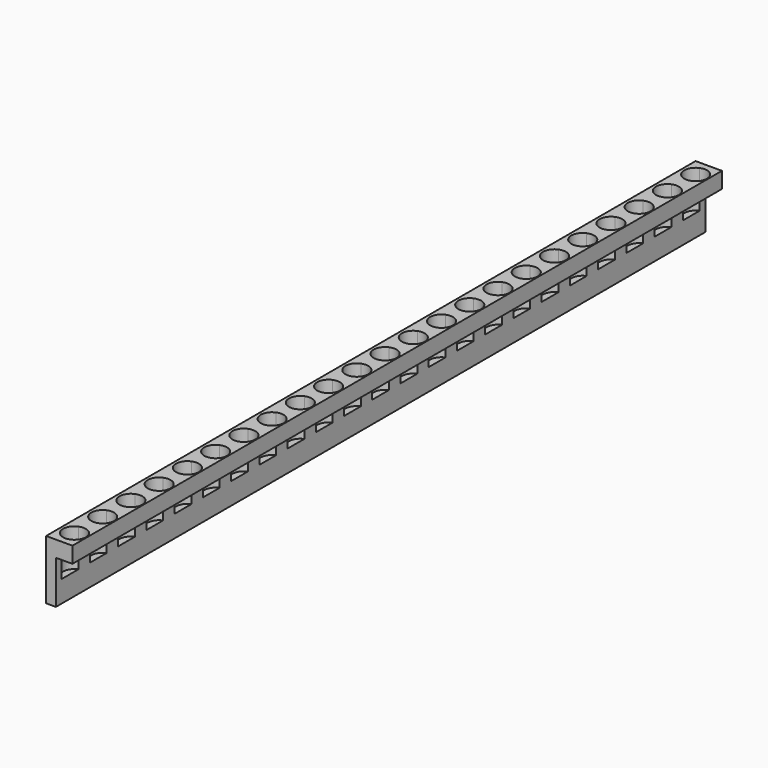
from build123d import *
from build123d import SkipClean  # not in build123d's __all__

# Parameters (mm, degrees)
F1_DEPTH = 4.318
F2_DEPTH = 4.318
F3_DEPTH = 5.842
F4_W     = 2.6416
F4_H     = 222.25
F5_DEPTH = 5.842
F6_DEPTH = 0.00508
F7_DEPTH = 3.19786


# Not quite as in the source:
# - after a boolean that leaves OpenCascade's solid faulty, fix() repairs it


with BuildPart() as f1:
    # F0 (on Top) → F1 (new body)
    with BuildSketch(Plane.XY):
        with BuildLine():
            Line((-21.6095393037, 173.5015366077), (-26.0799393037, 173.5015366077))
            Line((-26.0799393037, 173.5015366077), (-26.0799393037, 168.3720872764))
            ThreePointArc((-26.0799393037, 168.3720872764), (-23.1852887823, 168.1025078341), (-21.8103172985, 165.5410379171))
            ThreePointArc((-21.8103172985, 165.5410379171), (-23.1852887823, 162.9795680002), (-26.0799393037, 162.7099885579))
            Line((-26.0799393037, 162.7099885579), (-26.0799393037, 158.8512725119))
            ThreePointArc((-26.0799393037, 158.8512725119), (-23.1852887823, 158.5816930696), (-21.8103172985, 156.0202231526))
            ThreePointArc((-21.8103172985, 156.0202231526), (-23.1852887823, 153.4587532357), (-26.0799393037, 153.1891737934))
            Line((-26.0799393037, 153.1891737934), (-26.0799393037, 149.3262725119))
            ThreePointArc((-26.0799393037, 149.3262725119), (-23.1852887823, 149.0566930696), (-21.8103172985, 146.4952231526))
            ThreePointArc((-21.8103172985, 146.4952231526), (-23.1852887823, 143.9337532357), (-26.0799393037, 143.6641737934))
            Line((-26.0799393037, 143.6641737934), (-26.0799393037, 139.8012725119))
            ThreePointArc((-26.0799393037, 139.8012725119), (-23.1852887823, 139.5316930696), (-21.8103172985, 136.9702231526))
            ThreePointArc((-21.8103172985, 136.9702231526), (-23.1852887823, 134.4087532357), (-26.0799393037, 134.1391737934))
            Line((-26.0799393037, 134.1391737934), (-26.0799393037, 130.2762725119))
            ThreePointArc((-26.0799393037, 130.2762725119), (-23.1852887823, 130.0066930696), (-21.8103172985, 127.4452231526))
            ThreePointArc((-21.8103172985, 127.4452231526), (-23.1852887823, 124.8837532357), (-26.0799393037, 124.6141737934))
            Line((-26.0799393037, 124.6141737934), (-26.0799393037, 120.7512725119))
            ThreePointArc((-26.0799393037, 120.7512725119), (-23.1852887823, 120.4816930696), (-21.8103172985, 117.9202231526))
            ThreePointArc((-21.8103172985, 117.9202231526), (-23.1852887823, 115.3587532357), (-26.0799393037, 115.0891737934))
            Line((-26.0799393037, 115.0891737934), (-26.0799393037, 111.2262725119))
            ThreePointArc((-26.0799393037, 111.2262725119), (-23.1852887823, 110.9566930696), (-21.8103172985, 108.3952231526))
            ThreePointArc((-21.8103172985, 108.3952231526), (-23.1852887823, 105.8337532357), (-26.0799393037, 105.5641737934))
            Line((-26.0799393037, 105.5641737934), (-26.0799393037, 101.7012725119))
            ThreePointArc((-26.0799393037, 101.7012725119), (-23.1852887823, 101.4316930696), (-21.8103172985, 98.8702231526))
            ThreePointArc((-21.8103172985, 98.8702231526), (-23.1852887823, 96.3087532357), (-26.0799393037, 96.0391737934))
            Line((-26.0799393037, 96.0391737934), (-26.0799393037, 92.1762725119))
            ThreePointArc((-26.0799393037, 92.1762725119), (-23.1852887823, 91.9066930696), (-21.8103172985, 89.3452231526))
            ThreePointArc((-21.8103172985, 89.3452231526), (-23.1852887823, 86.7837532357), (-26.0799393037, 86.5141737934))
            Line((-26.0799393037, 86.5141737934), (-26.0799393037, 82.6512725119))
            ThreePointArc((-26.0799393037, 82.6512725119), (-23.1852887823, 82.3816930696), (-21.8103172985, 79.8202231526))
            ThreePointArc((-21.8103172985, 79.8202231526), (-23.1852887823, 77.2587532357), (-26.0799393037, 76.9891737934))
            Line((-26.0799393037, 76.9891737934), (-26.0799393037, 73.1374398831))
            ThreePointArc((-26.0799393037, 73.1374398831), (-23.1852887823, 72.8678604408), (-21.8103172985, 70.3063905239))
            ThreePointArc((-21.8103172985, 70.3063905239), (-23.1852887823, 67.744920607), (-26.0799393037, 67.4753411647))
            Line((-26.0799393037, 67.4753411647), (-26.0799393037, 63.6124425594))
            ThreePointArc((-26.0799393037, 63.6124425594), (-23.1852887823, 63.3428631171), (-21.8103172985, 60.7813932002))
            ThreePointArc((-21.8103172985, 60.7813932002), (-23.1852887823, 58.2199232832), (-26.0799393037, 57.9503438409))
            Line((-26.0799393037, 57.9503438409), (-26.0799393037, 54.0874415103))
            ThreePointArc((-26.0799393037, 54.0874415103), (-23.1852887823, 53.817862068), (-21.8103172985, 51.2563921511))
            ThreePointArc((-21.8103172985, 51.2563921511), (-23.1852887823, 48.6949222342), (-26.0799393037, 48.4253427919))
            Line((-26.0799393037, 48.4253427919), (-26.0799393037, 44.5624441866))
            ThreePointArc((-26.0799393037, 44.5624441866), (-23.1852887823, 44.2928647443), (-21.8103172985, 41.7313948274))
            ThreePointArc((-21.8103172985, 41.7313948274), (-23.1852887823, 39.1699249104), (-26.0799393037, 38.9003454681))
            Line((-26.0799393037, 38.9003454681), (-26.0799393037, 35.0374431376))
            ThreePointArc((-26.0799393037, 35.0374431376), (-23.1852887823, 34.7678636953), (-21.8103172985, 32.2063937783))
            ThreePointArc((-21.8103172985, 32.2063937783), (-23.1852887823, 29.6449238614), (-26.0799393037, 29.3753444191))
            Line((-26.0799393037, 29.3753444191), (-26.0799393037, 25.5124439512))
            ThreePointArc((-26.0799393037, 25.5124439512), (-23.1852887823, 25.2428645089), (-21.8103172985, 22.6813945919))
            ThreePointArc((-21.8103172985, 22.6813945919), (-23.1852887823, 20.119924675), (-26.0799393037, 19.8503452327))
            Line((-26.0799393037, 19.8503452327), (-26.0799393037, 15.9874438334))
            ThreePointArc((-26.0799393037, 15.9874438334), (-23.1852887823, 15.7178643911), (-21.8103172985, 13.1563944742))
            ThreePointArc((-21.8103172985, 13.1563944742), (-23.1852887823, 10.5949245573), (-26.0799393037, 10.325345115))
            Line((-26.0799393037, 10.325345115), (-26.0799393037, 6.4624434829))
            ThreePointArc((-26.0799393037, 6.4624434829), (-23.1852887823, 6.1928640406), (-21.8103172985, 3.6313941237))
            ThreePointArc((-21.8103172985, 3.6313941237), (-23.1852887823, 1.0699242067), (-26.0799393037, 0.8003447644))
            Line((-26.0799393037, 0.8003447644), (-26.0799393037, -3.0625568677))
            ThreePointArc((-26.0799393037, -3.0625568677), (-23.1852887823, -3.33213631), (-21.8103172985, -5.8936062269))
            ThreePointArc((-21.8103172985, -5.8936062269), (-23.1852887823, -8.4550761438), (-26.0799393037, -8.7246555861))
            Line((-26.0799393037, -8.7246555861), (-26.0799393037, -12.5809180524))
            ThreePointArc((-26.0799393037, -12.5809180524), (-23.1852887823, -12.8504974947), (-21.8103172985, -15.4119674116))
            ThreePointArc((-21.8103172985, -15.4119674116), (-23.1852887823, -17.9734373286), (-26.0799393037, -18.2430167709))
            Line((-26.0799393037, -18.2430167709), (-26.0799393037, -22.1085814592))
            ThreePointArc((-26.0799393037, -22.1085814592), (-23.1860931255, -22.3777536514), (-21.8114210892, -24.9384324998))
            ThreePointArc((-21.8114210892, -24.9384324998), (-23.1860931255, -27.4991113482), (-26.0799393037, -27.7682835404))
            Line((-26.0799393037, -27.7682835404), (-26.0799393037, -31.6266121611))
            ThreePointArc((-26.0799393037, -31.6266121611), (-23.1857640907, -31.8959509553), (-21.8109695623, -34.4569534063))
            ThreePointArc((-21.8109695623, -34.4569534063), (-23.1857640907, -37.0179558574), (-26.0799393037, -37.2872946516))
            Line((-26.0799393037, -37.2872946516), (-26.0799393037, -41.149786583))
            ThreePointArc((-26.0799393037, -41.149786583), (-23.1818467711, -41.4211080967), (-21.8055935227, -43.9859633923))
            ThreePointArc((-21.8055935227, -43.9859633923), (-23.1818467711, -46.5508186878), (-26.0799393037, -46.8221402015))
            Line((-26.0799393037, -46.8221402015), (-26.0799393037, -47.7885268629))
            Line((-26.0799393037, -47.7885268629), (-26.0799393037, -48.7484633923))
            Line((-26.0799393037, -48.7484633923), (-21.6095393037, -48.7484633923))
            Line((-21.6095393037, -48.7484633923), (-21.6095393037, 173.5015366077))
        make_face()
    extrude(amount=F1_DEPTH)

    # F0 (on Top) → F2 (join)
    with BuildSketch(Plane.XY):
        with BuildLine():
            Line((-26.0799393037, 173.5015366077), (-28.7215393037, 173.5015366077))
            Line((-28.7215393037, 173.5015366077), (-28.7215393037, -48.7484633923))
            Line((-28.7215393037, -48.7484633923), (-26.0799393037, -48.7484633923))
            Line((-26.0799393037, -48.7484633923), (-26.0799393037, -47.7885268629))
            Line((-26.0799393037, -47.7885268629), (-26.0799393037, -46.8221402015))
            ThreePointArc((-26.0799393037, -46.8221402015), (-27.9618410743, -43.9859633923), (-26.0799393037, -41.149786583))
            Line((-26.0799393037, -41.149786583), (-26.0799393037, -37.2872946516))
            ThreePointArc((-26.0799393037, -37.2872946516), (-27.9564650347, -34.4569534063), (-26.0799393037, -31.6266121611))
            Line((-26.0799393037, -31.6266121611), (-26.0799393037, -27.7682835404))
            ThreePointArc((-26.0799393037, -27.7682835404), (-27.9560135078, -24.9384324998), (-26.0799393037, -22.1085814592))
            Line((-26.0799393037, -22.1085814592), (-26.0799393037, -18.2430167709))
            ThreePointArc((-26.0799393037, -18.2430167709), (-27.9571172985, -15.4119674116), (-26.0799393037, -12.5809180524))
            Line((-26.0799393037, -12.5809180524), (-26.0799393037, -8.7246555861))
            ThreePointArc((-26.0799393037, -8.7246555861), (-27.9571172985, -5.8936062269), (-26.0799393037, -3.0625568677))
            Line((-26.0799393037, -3.0625568677), (-26.0799393037, 0.8003447644))
            ThreePointArc((-26.0799393037, 0.8003447644), (-27.9571172985, 3.6313941237), (-26.0799393037, 6.4624434829))
            Line((-26.0799393037, 6.4624434829), (-26.0799393037, 10.325345115))
            ThreePointArc((-26.0799393037, 10.325345115), (-27.9571172985, 13.1563944742), (-26.0799393037, 15.9874438334))
            Line((-26.0799393037, 15.9874438334), (-26.0799393037, 19.8503452327))
            ThreePointArc((-26.0799393037, 19.8503452327), (-27.9571172985, 22.6813945919), (-26.0799393037, 25.5124439512))
            Line((-26.0799393037, 25.5124439512), (-26.0799393037, 29.3753444191))
            ThreePointArc((-26.0799393037, 29.3753444191), (-27.9571172985, 32.2063937783), (-26.0799393037, 35.0374431376))
            Line((-26.0799393037, 35.0374431376), (-26.0799393037, 38.9003454681))
            ThreePointArc((-26.0799393037, 38.9003454681), (-27.9571172985, 41.7313948274), (-26.0799393037, 44.5624441866))
            Line((-26.0799393037, 44.5624441866), (-26.0799393037, 48.4253427919))
            ThreePointArc((-26.0799393037, 48.4253427919), (-27.9571172985, 51.2563921511), (-26.0799393037, 54.0874415103))
            Line((-26.0799393037, 54.0874415103), (-26.0799393037, 57.9503438409))
            ThreePointArc((-26.0799393037, 57.9503438409), (-27.9571172985, 60.7813932002), (-26.0799393037, 63.6124425594))
            Line((-26.0799393037, 63.6124425594), (-26.0799393037, 67.4753411647))
            ThreePointArc((-26.0799393037, 67.4753411647), (-27.9571172985, 70.3063905239), (-26.0799393037, 73.1374398831))
            Line((-26.0799393037, 73.1374398831), (-26.0799393037, 76.9891737934))
            ThreePointArc((-26.0799393037, 76.9891737934), (-27.9571172985, 79.8202231526), (-26.0799393037, 82.6512725119))
            Line((-26.0799393037, 82.6512725119), (-26.0799393037, 86.5141737934))
            ThreePointArc((-26.0799393037, 86.5141737934), (-27.9571172985, 89.3452231526), (-26.0799393037, 92.1762725119))
            Line((-26.0799393037, 92.1762725119), (-26.0799393037, 96.0391737934))
            ThreePointArc((-26.0799393037, 96.0391737934), (-27.9571172985, 98.8702231526), (-26.0799393037, 101.7012725119))
            Line((-26.0799393037, 101.7012725119), (-26.0799393037, 105.5641737934))
            ThreePointArc((-26.0799393037, 105.5641737934), (-27.9571172985, 108.3952231526), (-26.0799393037, 111.2262725119))
            Line((-26.0799393037, 111.2262725119), (-26.0799393037, 115.0891737934))
            ThreePointArc((-26.0799393037, 115.0891737934), (-27.9571172985, 117.9202231526), (-26.0799393037, 120.7512725119))
            Line((-26.0799393037, 120.7512725119), (-26.0799393037, 124.6141737934))
            ThreePointArc((-26.0799393037, 124.6141737934), (-27.9571172985, 127.4452231526), (-26.0799393037, 130.2762725119))
            Line((-26.0799393037, 130.2762725119), (-26.0799393037, 134.1391737934))
            ThreePointArc((-26.0799393037, 134.1391737934), (-27.9571172985, 136.9702231526), (-26.0799393037, 139.8012725119))
            Line((-26.0799393037, 139.8012725119), (-26.0799393037, 143.6641737934))
            ThreePointArc((-26.0799393037, 143.6641737934), (-27.9571172985, 146.4952231526), (-26.0799393037, 149.3262725119))
            Line((-26.0799393037, 149.3262725119), (-26.0799393037, 153.1891737934))
            ThreePointArc((-26.0799393037, 153.1891737934), (-27.9571172985, 156.0202231526), (-26.0799393037, 158.8512725119))
            Line((-26.0799393037, 158.8512725119), (-26.0799393037, 162.7099885579))
            ThreePointArc((-26.0799393037, 162.7099885579), (-27.9571172985, 165.5410379171), (-26.0799393037, 168.3720872764))
            Line((-26.0799393037, 168.3720872764), (-26.0799393037, 173.5015366077))
        make_face()
    extrude(amount=F2_DEPTH)

    # F0 (on Top) → F3 (join)
    with BuildSketch(Plane.XY):
        with BuildLine():
            Line((-26.0799393037, 173.5015366077), (-28.7215393037, 173.5015366077))
            Line((-28.7215393037, 173.5015366077), (-28.7215393037, -48.7484633923))
            Line((-28.7215393037, -48.7484633923), (-26.0799393037, -48.7484633923))
            Line((-26.0799393037, -48.7484633923), (-26.0799393037, -47.7885268629))
            Line((-26.0799393037, -47.7885268629), (-26.0799393037, -46.8221402015))
            ThreePointArc((-26.0799393037, -46.8221402015), (-27.9618410743, -43.9859633923), (-26.0799393037, -41.149786583))
            Line((-26.0799393037, -41.149786583), (-26.0799393037, -37.2872946516))
            ThreePointArc((-26.0799393037, -37.2872946516), (-27.9564650347, -34.4569534063), (-26.0799393037, -31.6266121611))
            Line((-26.0799393037, -31.6266121611), (-26.0799393037, -27.7682835404))
            ThreePointArc((-26.0799393037, -27.7682835404), (-27.9560135078, -24.9384324998), (-26.0799393037, -22.1085814592))
            Line((-26.0799393037, -22.1085814592), (-26.0799393037, -18.2430167709))
            ThreePointArc((-26.0799393037, -18.2430167709), (-27.9571172985, -15.4119674116), (-26.0799393037, -12.5809180524))
            Line((-26.0799393037, -12.5809180524), (-26.0799393037, -8.7246555861))
            ThreePointArc((-26.0799393037, -8.7246555861), (-27.9571172985, -5.8936062269), (-26.0799393037, -3.0625568677))
            Line((-26.0799393037, -3.0625568677), (-26.0799393037, 0.8003447644))
            ThreePointArc((-26.0799393037, 0.8003447644), (-27.9571172985, 3.6313941237), (-26.0799393037, 6.4624434829))
            Line((-26.0799393037, 6.4624434829), (-26.0799393037, 10.325345115))
            ThreePointArc((-26.0799393037, 10.325345115), (-27.9571172985, 13.1563944742), (-26.0799393037, 15.9874438334))
            Line((-26.0799393037, 15.9874438334), (-26.0799393037, 19.8503452327))
            ThreePointArc((-26.0799393037, 19.8503452327), (-27.9571172985, 22.6813945919), (-26.0799393037, 25.5124439512))
            Line((-26.0799393037, 25.5124439512), (-26.0799393037, 29.3753444191))
            ThreePointArc((-26.0799393037, 29.3753444191), (-27.9571172985, 32.2063937783), (-26.0799393037, 35.0374431376))
            Line((-26.0799393037, 35.0374431376), (-26.0799393037, 38.9003454681))
            ThreePointArc((-26.0799393037, 38.9003454681), (-27.9571172985, 41.7313948274), (-26.0799393037, 44.5624441866))
            Line((-26.0799393037, 44.5624441866), (-26.0799393037, 48.4253427919))
            ThreePointArc((-26.0799393037, 48.4253427919), (-27.9571172985, 51.2563921511), (-26.0799393037, 54.0874415103))
            Line((-26.0799393037, 54.0874415103), (-26.0799393037, 57.9503438409))
            ThreePointArc((-26.0799393037, 57.9503438409), (-27.9571172985, 60.7813932002), (-26.0799393037, 63.6124425594))
            Line((-26.0799393037, 63.6124425594), (-26.0799393037, 67.4753411647))
            ThreePointArc((-26.0799393037, 67.4753411647), (-27.9571172985, 70.3063905239), (-26.0799393037, 73.1374398831))
            Line((-26.0799393037, 73.1374398831), (-26.0799393037, 76.9891737934))
            ThreePointArc((-26.0799393037, 76.9891737934), (-27.9571172985, 79.8202231526), (-26.0799393037, 82.6512725119))
            Line((-26.0799393037, 82.6512725119), (-26.0799393037, 86.5141737934))
            ThreePointArc((-26.0799393037, 86.5141737934), (-27.9571172985, 89.3452231526), (-26.0799393037, 92.1762725119))
            Line((-26.0799393037, 92.1762725119), (-26.0799393037, 96.0391737934))
            ThreePointArc((-26.0799393037, 96.0391737934), (-27.9571172985, 98.8702231526), (-26.0799393037, 101.7012725119))
            Line((-26.0799393037, 101.7012725119), (-26.0799393037, 105.5641737934))
            ThreePointArc((-26.0799393037, 105.5641737934), (-27.9571172985, 108.3952231526), (-26.0799393037, 111.2262725119))
            Line((-26.0799393037, 111.2262725119), (-26.0799393037, 115.0891737934))
            ThreePointArc((-26.0799393037, 115.0891737934), (-27.9571172985, 117.9202231526), (-26.0799393037, 120.7512725119))
            Line((-26.0799393037, 120.7512725119), (-26.0799393037, 124.6141737934))
            ThreePointArc((-26.0799393037, 124.6141737934), (-27.9571172985, 127.4452231526), (-26.0799393037, 130.2762725119))
            Line((-26.0799393037, 130.2762725119), (-26.0799393037, 134.1391737934))
            ThreePointArc((-26.0799393037, 134.1391737934), (-27.9571172985, 136.9702231526), (-26.0799393037, 139.8012725119))
            Line((-26.0799393037, 139.8012725119), (-26.0799393037, 143.6641737934))
            ThreePointArc((-26.0799393037, 143.6641737934), (-27.9571172985, 146.4952231526), (-26.0799393037, 149.3262725119))
            Line((-26.0799393037, 149.3262725119), (-26.0799393037, 153.1891737934))
            ThreePointArc((-26.0799393037, 153.1891737934), (-27.9571172985, 156.0202231526), (-26.0799393037, 158.8512725119))
            Line((-26.0799393037, 158.8512725119), (-26.0799393037, 162.7099885579))
            ThreePointArc((-26.0799393037, 162.7099885579), (-27.9571172985, 165.5410379171), (-26.0799393037, 168.3720872764))
            Line((-26.0799393037, 168.3720872764), (-26.0799393037, 173.5015366077))
        make_face()
    with SkipClean():  # cleaning this boolean's faces spoils the solid; the shape is the same uncleaned
        extrude(amount=-F3_DEPTH)

    # F4 (on face) → F5 (join)
    with BuildSketch(Plane(origin=(0, 0, -5.842), x_dir=(1, 0, 0), z_dir=(0, 0, -1))):
        with Locations((-27.4007393037, -62.3765366077)):
            Rectangle(F4_W, F4_H)
    extrude(amount=F5_DEPTH)

    add(f1.part.fix(), mode=Mode.REPLACE)

    # F6 (add): faces of the model
    f6_faces = [f1.faces().sort_by_distance(p)[0] for p in [
        (-25.1655393037, -48.7484633923, 2.159),
        (-27.4007393037, -48.7484633923, -2.921),
        (-27.4007393037, -48.7484633923, -8.763),
    ]]
    extrude(f6_faces, amount=F6_DEPTH)

    add(f1.part.fix(), mode=Mode.REPLACE)

    # F7 (cut): faces of the model
    f7_faces = [f1.faces().sort_by_distance(p)[0] for p in [
        (-25.1655393037, 173.5015366077, 2.159),
        (-27.4007393037, 173.5015366077, -2.921),
        (-27.4007393037, 173.5015366077, -8.763),
    ]]
    extrude(f7_faces, amount=-F7_DEPTH, mode=Mode.SUBTRACT)

    add(f1.part.fix(), mode=Mode.REPLACE)


solid = f1.part
